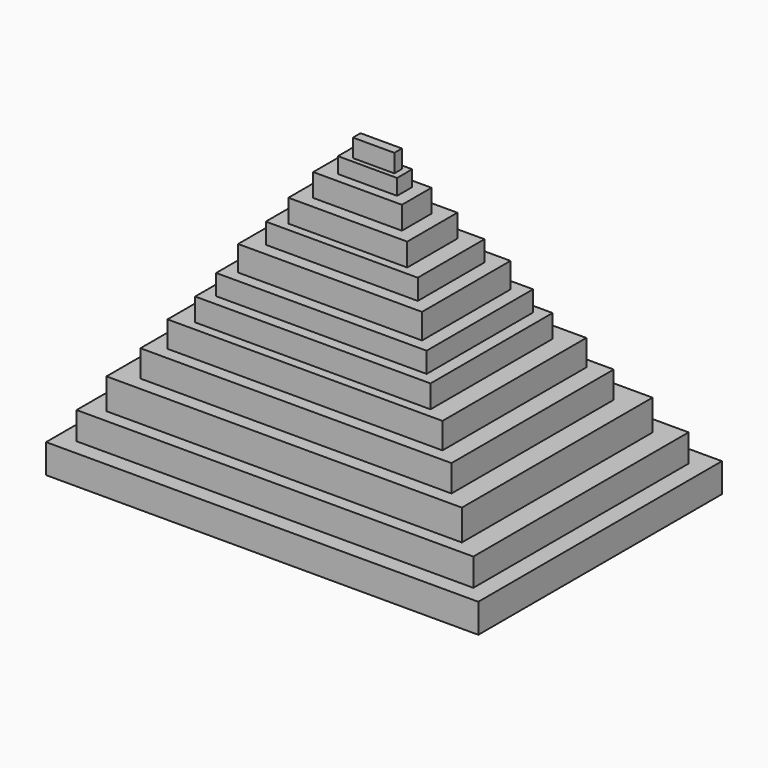
from build123d import *

# Parameters (mm, degrees)
F0_W      = 13.366825413
F0_H      = 3.0552744865
F1_DEPTH  = 99.568
F0_W_2    = 19.0954655409
F0_H_2    = 6.1105492059
F2_DEPTH  = 93.726
F0_W_3    = 28.6431992427
F0_H_3    = 11.9346659631
F3_DEPTH  = 88.646
F0_W_4    = 38.3818857372
F0_H_4    = 20.2411934733
F4_DEPTH  = 81.28
F0_W_5    = 49.0753464401
F0_H_5    = 26.9246064126
F5_DEPTH  = 73.914
F0_W_6    = 59.3868978322
F0_H_6    = 35.7085214928
F6_DEPTH  = 67.31
F0_W_7    = 67.9798536003
F0_H_7    = 42.964797467
F7_DEPTH  = 59.182
F0_W_8    = 75.9999491274
F0_H_8    = 49.2663010955
F8_DEPTH  = 52.578
F0_W_9    = 88.7939184904
F0_H_9    = 58.0502152443
F9_DEPTH  = 45.212
F0_W_10   = 100.4421524704
F0_H_10   = 65.4974486679
F10_DEPTH = 36.83
F0_W_11   = 114.7637441754
F0_H_11   = 76.9547224045
F11_DEPTH = 28.194
F0_W_12   = 128.1305700541
F0_H_12   = 86.884368211
F12_DEPTH = 18.288
F0_W_13   = 139.5878568292
F0_H_13   = 98.3416512609
F13_DEPTH = 9.398


# Not quite as in the source:
# - the program builds the solid bodies; features that only make, move or delete a surface that nothing else refers to are left out


with BuildPart() as f1:
    # F0 (on Top) → F1 (new body)
    with BuildSketch(Plane.XY):
        with Locations((1.8140685279, -5.8241172228)):
            Rectangle(F0_W, F0_H)
    extrude(amount=F1_DEPTH)

    # F0 (on Top) → F2 (join)
    with BuildSketch(Plane.XY):
        with Locations((1.0502506047, -5.8241168736)):
            Rectangle(F0_W_2, F0_H_2)
        with Locations((1.8140685279, -5.8241172228)):
            Rectangle(F0_W, F0_H, mode=Mode.SUBTRACT)
    extrude(amount=F2_DEPTH)

    # F0 (on Top) → F3 (join)
    with BuildSketch(Plane.XY):
        with Locations((0.2864324488, -5.9673329815)):
            Rectangle(F0_W_3, F0_H_3)
        with Locations((1.0502506047, -5.8241168736)):
            Rectangle(F0_W_2, F0_H_2, mode=Mode.SUBTRACT)
    extrude(amount=F3_DEPTH)

    # F0 (on Top) → F4 (join)
    with BuildSketch(Plane.XY):
        with Locations((0.1909546554, -5.6331623346)):
            Rectangle(F0_W_4, F0_H_4)
        with Locations((0.2864324488, -5.9673329815)):
            Rectangle(F0_W_3, F0_H_3, mode=Mode.SUBTRACT)
    extrude(amount=F4_DEPTH)

    # F0 (on Top) → F5 (join)
    with BuildSketch(Plane.XY):
        with Locations((0.3819093108, -4.9648210406)):
            Rectangle(F0_W_5, F0_H_5)
        with Locations((0.1909546554, -5.6331623346)):
            Rectangle(F0_W_4, F0_H_4, mode=Mode.SUBTRACT)
    extrude(amount=F5_DEPTH)

    # F0 (on Top) → F6 (join)
    with BuildSketch(Plane.XY):
        with Locations((-0.1909546554, -4.5829112642)):
            Rectangle(F0_W_6, F0_H_6)
        with Locations((0.3819093108, -4.9648210406)):
            Rectangle(F0_W_5, F0_H_5, mode=Mode.SUBTRACT)
    extrude(amount=F6_DEPTH)

    # F0 (on Top) → F7 (join)
    with BuildSketch(Plane.XY):
        with Locations((-0.0954773277, -4.5829117298)):
            Rectangle(F0_W_7, F0_H_7)
        with Locations((-0.1909546554, -4.5829112642)):
            Rectangle(F0_W_6, F0_H_6, mode=Mode.SUBTRACT)
    extrude(amount=F7_DEPTH)

    # F0 (on Top) → F8 (join)
    with BuildSketch(Plane.XY):
        with Locations((-0.0954773277, -4.8693437129)):
            Rectangle(F0_W_8, F0_H_8)
        with Locations((-0.0954773277, -4.5829117298)):
            Rectangle(F0_W_7, F0_H_7, mode=Mode.SUBTRACT)
    extrude(amount=F8_DEPTH)

    # F0 (on Top) → F9 (join)
    with BuildSketch(Plane.XY):
        with Locations((-0.1909546554, -3.5326592624)):
            Rectangle(F0_W_9, F0_H_9)
        with Locations((-0.0954773277, -4.8693437129)):
            Rectangle(F0_W_8, F0_H_8, mode=Mode.SUBTRACT)
    extrude(amount=F9_DEPTH)

    # F0 (on Top) → F10 (join)
    with BuildSketch(Plane.XY):
        with Locations((0.0954773277, -3.8190940395)):
            Rectangle(F0_W_10, F0_H_10)
        with Locations((-0.1909546554, -3.5326592624)):
            Rectangle(F0_W_9, F0_H_9, mode=Mode.SUBTRACT)
    extrude(amount=F10_DEPTH)

    # F0 (on Top) → F11 (join)
    with BuildSketch(Plane.XY):
        with Locations((-0.1909546554, -2.4824105203)):
            Rectangle(F0_W_11, F0_H_11)
        with Locations((0.0954773277, -3.8190940395)):
            Rectangle(F0_W_10, F0_H_10, mode=Mode.SUBTRACT)
    extrude(amount=F11_DEPTH)

    # F0 (on Top) → F12 (join)
    with BuildSketch(Plane.XY):
        with Locations((0.1909509301, -1.718590036)):
            Rectangle(F0_W_12, F0_H_12)
        with Locations((-0.1909546554, -2.4824105203)):
            Rectangle(F0_W_11, F0_H_11, mode=Mode.SUBTRACT)
    extrude(amount=F12_DEPTH)

    # F0 (on Top) → F13 (join)
    with BuildSketch(Plane.XY):
        with Locations((0.1909546554, -1.1457279325)):
            Rectangle(F0_W_13, F0_H_13)
        with Locations((0.1909509301, -1.718590036)):
            Rectangle(F0_W_12, F0_H_12, mode=Mode.SUBTRACT)
    extrude(amount=F13_DEPTH)


solid = f1.part
